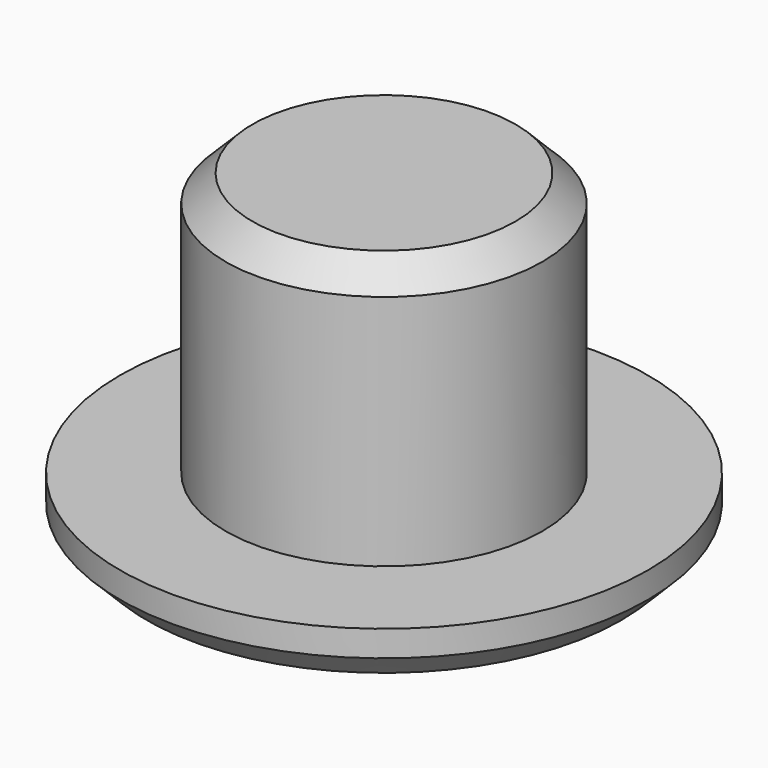
from build123d import *

# Parameters (mm, degrees)
F0_R      = 15
F1_DEPTH  = 25
F0_R_2    = 25
F1_FACE_R = 15
F2_DEPTH  = 5
F3_SIZE   = 2.54
F4_SIZE   = 2.54


with BuildPart() as f1:
    # F0 (on Top) → F1 (new body)
    with BuildSketch(Plane.XY):
        Circle(F0_R)
    extrude(amount=F1_DEPTH)

    # F0 (on Top) + F1_face (on face) → F2 (join)
    with BuildSketch(Plane.XY):
        Circle(F0_R_2)
        Circle(F0_R, mode=Mode.SUBTRACT)
    with BuildSketch(Plane.XY.offset(25)):
        Circle(F1_FACE_R)
    extrude(amount=F2_DEPTH)

    # F3
    f3_edges = [f1.edges().sort_by_distance(p)[0] for p in [
        (-25, 0, 0),
    ]]
    chamfer(f3_edges, length=F3_SIZE)

    # F4
    f4_edges = [f1.edges().sort_by_distance(p)[0] for p in [
        (-15, 0, 30),
    ]]
    chamfer(f4_edges, length=F4_SIZE)


solid = f1.part
